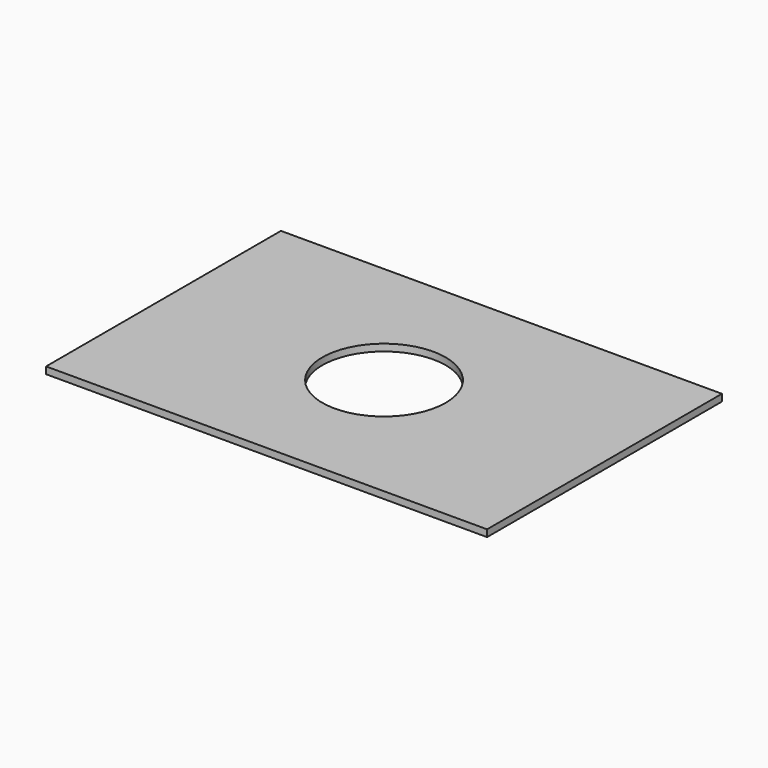
from build123d import *

# Parameters (mm, degrees)
F2_W     = 127.7
F2_H     = 85
F2_R     = 17.85
F3_DEPTH = 2


# Not quite as in the source:
# - a feature names something its author has since deleted; it is built from what else it names


with BuildPart() as f3:
    # F2 (on offset) → F3 (new body)
    with BuildSketch(Plane.XY.offset(2)):
        Rectangle(F2_W, F2_H)
        Circle(F2_R, mode=Mode.SUBTRACT)
    extrude(amount=-F3_DEPTH)


solid = f3.part
